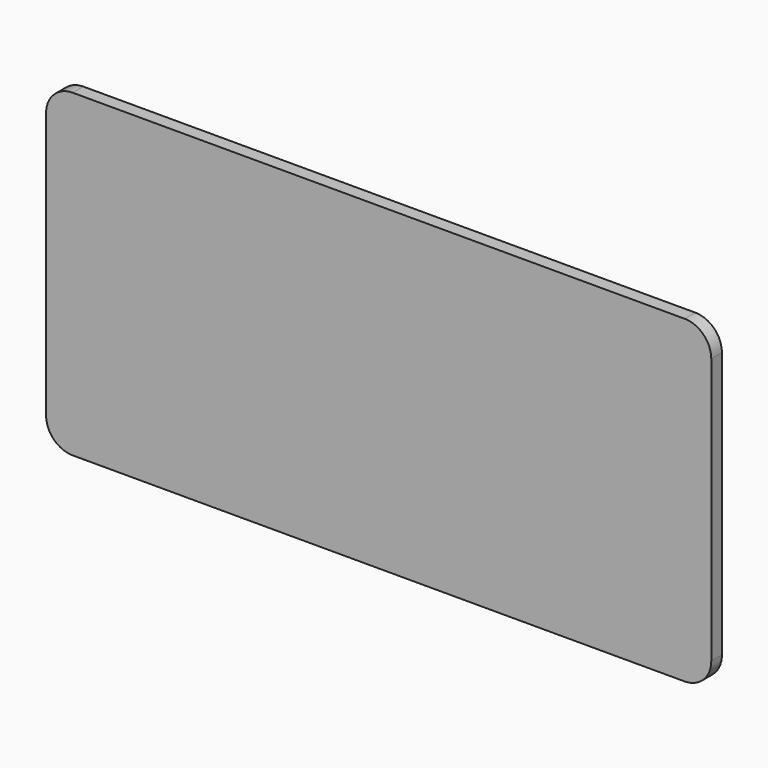
from build123d import *

# Parameters (mm, degrees)
F0_W         = 6350
F0_H         = 3048
F1_DEPTH     = 127
F2_TEXT_SIZE = 683.7371760876
F3_DEPTH     = 76.2
F4_TEXT_SIZE = 557.7492402706
F5_DEPTH     = 76.2
F6_R         = 254
F7_TEXT_SIZE = 301.742499826
F8_DEPTH     = 76.2
F9_TEXT_SIZE = 257.7644347661
F10_DEPTH    = 76.2


# Not quite as in the source:
# - Text() gives the source's letters only with a copy of the font that has no kerning and outlines rounded to 1/6400 em; it was checked with that copy


with BuildPart() as f1:
    # F0 (on Front) → F1 (new body)
    with BuildSketch(Plane.XZ):
        Rectangle(F0_W, F0_H)
    extrude(amount=F1_DEPTH)

    # F2 (on face) → F3 (cut)
    with BuildSketch(Plane(origin=(0, 0, 0), x_dir=(-1, 0, 0), z_dir=(0, 1, 0))):
        with Locations((-2921, 523.7092332169)):
            Text('TEDx Alessandria', F2_TEXT_SIZE, font='Open Sans', font_style=FontStyle.BOLD, text_align=(TextAlign.LEFT, TextAlign.BOTTOM))
    extrude(amount=-F3_DEPTH, mode=Mode.SUBTRACT)

    # F4 (on face) → F5 (cut)
    with BuildSketch(Plane(origin=(0, 0, 0), x_dir=(-1, 0, 0), z_dir=(0, 1, 0))):
        with Locations((-889, -1016)):
            Text('Grazie', F4_TEXT_SIZE, font='Open Sans', font_style=FontStyle.BOLD, text_align=(TextAlign.LEFT, TextAlign.BOTTOM))
    extrude(amount=-F5_DEPTH, mode=Mode.SUBTRACT)

    # F6
    f6_edges = [f1.edges().sort_by_distance(p)[0] for p in [
        (-3175, -63.5, 1524),
        (3175, -63.5, 1524),
        (3175, -63.5, -1524),
        (-3175, -63.5, -1524),
    ]]
    fillet(f6_edges, radius=F6_R)

    # F7 (on face) → F8 (cut)
    with BuildSketch(Plane(origin=(0, 0, 0), x_dir=(-1, 0, 0), z_dir=(0, 1, 0))):
        with Locations((-1016, 163.7454001253)):
            Text('Edizione 2017', F7_TEXT_SIZE, font='Open Sans', font_style=FontStyle.BOLD, text_align=(TextAlign.LEFT, TextAlign.BOTTOM))
    extrude(amount=-F8_DEPTH, mode=Mode.SUBTRACT)

    # F9 (on face) → F10 (cut)
    with BuildSketch(Plane(origin=(0, 0, 0), x_dir=(-1, 0, 0), z_dir=(0, 1, 0))):
        with Locations((-1905, -185.5903930316)):
            Text('Nuove forme e nuovi percorsi', F9_TEXT_SIZE, font='Open Sans', font_style=FontStyle.BOLD, text_align=(TextAlign.LEFT, TextAlign.BOTTOM))
    extrude(amount=-F10_DEPTH, mode=Mode.SUBTRACT)


solid = f1.part
